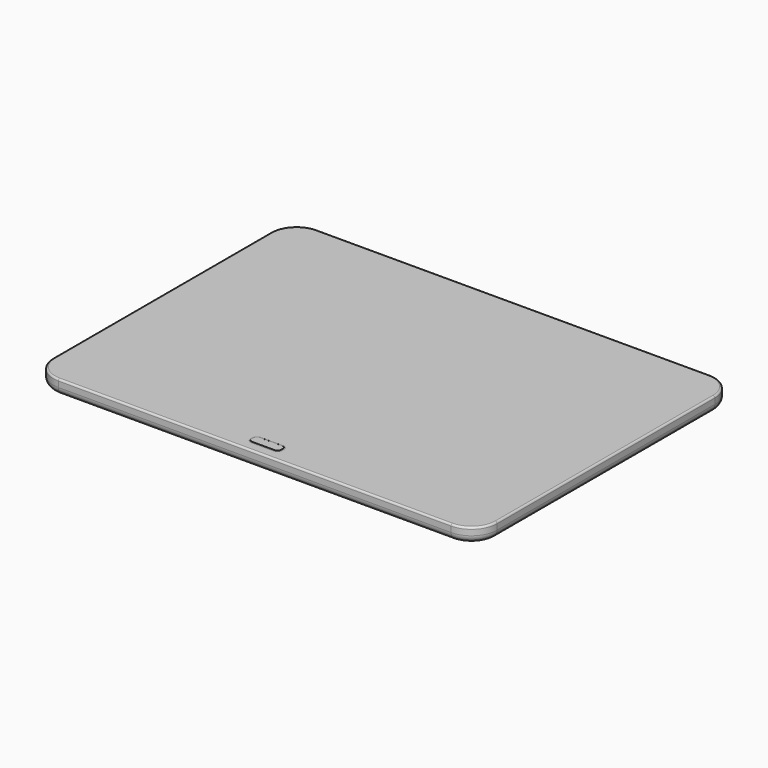
from build123d import *

# Parameters (mm, degrees)
F0_W         = 243
F0_H         = 177
F1_DEPTH     = 8.1
F2_R         = 14
F3_W         = 16.2
F3_H         = 5.2
F4_DEPTH     = 0.2
F5_R         = 2
F6_R         = 4
F7_T1_DEPTH  = 12.2
F7_T3_DEPTH  = 1.2
F7_T6_ANGLE  = 90
F7_T8_ANGLE  = 90
F7_T10_ANGLE = 90
F7_T12_ANGLE = 90
F7_T13_DEPTH = 215
F7_T15_DEPTH = 149
F7_T18_ANGLE = 90
F7_T20_ANGLE = 90
F7_T22_ANGLE = 90
F7_T24_ANGLE = 90


# Not quite as in the source:
# - a fillet or chamfer that OpenCascade refuses, or shapes differently, is made with other operations: its cross-section is extruded or revolved along the edge and cut away or added


with BuildPart() as f1:
    # F0 (on Top) → F1 (new body)
    with BuildSketch(Plane.XY):
        with Locations((0, 88.5)):
            Rectangle(F0_W, F0_H)
    extrude(amount=F1_DEPTH)

    # F2
    f2_edges = [f1.edges().sort_by_distance(p)[0] for p in [
        (-121.5, 0, 4.05),
        (121.5, 0, 4.05),
        (121.5, 177, 4.05),
        (-121.5, 177, 4.05),
    ]]
    fillet(f2_edges, radius=F2_R)

    # F3 (on face) → F4 (join)
    with BuildSketch(Plane.XY.offset(8.1)):
        with Locations((0, 8.6)):
            Rectangle(F3_W, F3_H)
    extrude(amount=F4_DEPTH)

    # F5
    f5_edges = [f1.edges().sort_by_distance(p)[0] for p in [
        (8.1, 6, 8.2),
        (8.1, 11.2, 8.2),
        (-8.1, 6, 8.2),
        (-8.1, 11.2, 8.2),
    ]]
    fillet(f5_edges, radius=F5_R)

    # F6
    f6_edges = [f1.edges().sort_by_distance(p)[0] for p in [
        (121.5, 88.5, 0),
        (0, 177, 0),
        (117.399495, 172.899495, 0),
        (-117.399495, 172.899495, 0),
        (-121.5, 88.5, 0),
        (117.399495, 4.100505, 0),
        (-117.399495, 4.100505, 0),
        (0, 0, 0),
    ]]
    fillet(f6_edges, radius=F6_R)

    # F7: fillet of radius 1 on 16 edges, made by hand

    # F7_s2 → F7_t1 (join)
    with BuildSketch(Plane.YZ.offset(-6.1)):
        with BuildLine():
            ThreePointArc((11.8, 8.1), (11.483772234, 8.1513167019), (11.2, 8.3))
            Line((11.2, 8.3), (11.2, 8.1))
            Line((11.2, 8.1), (11.8, 8.1))
        make_face()
        with BuildLine():
            ThreePointArc((5.4, 8.1), (5.716227766, 8.1513167019), (6, 8.3))
            Line((6, 8.3), (6, 8.1))
            Line((6, 8.1), (5.4, 8.1))
        make_face()
    extrude(amount=F7_T1_DEPTH)

    # F7_s4 → F7_t3 (join)
    with BuildSketch(Plane.XZ.offset(-9.2)):
        with BuildLine():
            ThreePointArc((8.7, 8.1), (8.383772234, 8.1513167019), (8.1, 8.3))
            Line((8.1, 8.3), (8.1, 8.1))
            Line((8.1, 8.1), (8.7, 8.1))
        make_face()
        with BuildLine():
            ThreePointArc((-8.7, 8.1), (-8.383772234, 8.1513167019), (-8.1, 8.3))
            Line((-8.1, 8.3), (-8.1, 8.1))
            Line((-8.1, 8.1), (-8.7, 8.1))
        make_face()
    extrude(amount=F7_T3_DEPTH)

    # F7_s5 → F7_t6 (revolve)
    with BuildSketch(Plane.YZ.offset(6.1)):
        with BuildLine():
            ThreePointArc((11.8, 8.1), (11.483772234, 8.1513167019), (11.2, 8.3))
            Line((11.2, 8.3), (11.2, 8.1))
            Line((11.2, 8.1), (11.8, 8.1))
        make_face()
    revolve(axis=Axis((6.1, 9.2, 8.1), (0, 0, -1)), revolution_arc=F7_T6_ANGLE)

    # F7_s7 → F7_t8 (revolve)
    with BuildSketch(Plane.YZ.offset(-6.1)):
        with BuildLine():
            ThreePointArc((11.8, 8.1), (11.483772234, 8.1513167019), (11.2, 8.3))
            Line((11.2, 8.3), (11.2, 8.1))
            Line((11.2, 8.1), (11.8, 8.1))
        make_face()
    revolve(axis=Axis((-6.1, 9.2, 8.1), (0, 0, 1)), revolution_arc=F7_T8_ANGLE)

    # F7_s9 → F7_t10 (revolve)
    with BuildSketch(Plane.YZ.offset(6.1)):
        with BuildLine():
            ThreePointArc((5.4, 8.1), (5.716227766, 8.1513167019), (6, 8.3))
            Line((6, 8.3), (6, 8.1))
            Line((6, 8.1), (5.4, 8.1))
        make_face()
    revolve(axis=Axis((6.1, 8, 8.1), (0, 0, 1)), revolution_arc=F7_T10_ANGLE)

    # F7_s11 → F7_t12 (revolve)
    with BuildSketch(Plane.XZ.offset(-8)):
        with BuildLine():
            ThreePointArc((-8.7, 8.1), (-8.383772234, 8.1513167019), (-8.1, 8.3))
            Line((-8.1, 8.3), (-8.1, 8.1))
            Line((-8.1, 8.1), (-8.7, 8.1))
        make_face()
    revolve(axis=Axis((-6.1, 8, 8.1), (0, 0, 1)), revolution_arc=F7_T12_ANGLE)

    # F7_s14 → F7_t13 (cut)
    with BuildSketch(Plane.YZ.offset(-107.5)):
        with BuildLine():
            ThreePointArc((177, 7.1), (176.7071067812, 7.8071067812), (176, 8.1))
            Line((176, 8.1), (177, 8.1))
            Line((177, 8.1), (177, 7.1))
        make_face()
        with BuildLine():
            ThreePointArc((1, 8.1), (0.2928932188, 7.8071067812), (0, 7.1))
            Line((0, 7.1), (0, 8.1))
            Line((0, 8.1), (1, 8.1))
        make_face()
    extrude(amount=F7_T13_DEPTH, mode=Mode.SUBTRACT)

    # F7_s16 → F7_t15 (cut)
    with BuildSketch(Plane.XZ.offset(-163)):
        with BuildLine():
            ThreePointArc((120.5, 8.1), (121.2071067812, 7.8071067812), (121.5, 7.1))
            Line((121.5, 7.1), (121.5, 8.1))
            Line((121.5, 8.1), (120.5, 8.1))
        make_face()
        with BuildLine():
            ThreePointArc((-120.5, 8.1), (-121.2071067812, 7.8071067812), (-121.5, 7.1))
            Line((-121.5, 7.1), (-121.5, 8.1))
            Line((-121.5, 8.1), (-120.5, 8.1))
        make_face()
    extrude(amount=F7_T15_DEPTH, mode=Mode.SUBTRACT)

    # F7_s17 → F7_t18 (revolve, cut)
    with BuildSketch(Plane.YZ.offset(107.5)):
        with BuildLine():
            ThreePointArc((177, 7.1), (176.7071067812, 7.8071067812), (176, 8.1))
            Line((176, 8.1), (177, 8.1))
            Line((177, 8.1), (177, 7.1))
        make_face()
    revolve(axis=Axis((107.5, 163, 8.1), (0, 0, -1)), revolution_arc=F7_T18_ANGLE, mode=Mode.SUBTRACT)

    # F7_s19 → F7_t20 (revolve, cut)
    with BuildSketch(Plane.YZ.offset(-107.5)):
        with BuildLine():
            ThreePointArc((176, 8.1), (176.7071067812, 7.8071067812), (177, 7.1))
            Line((177, 7.1), (177, 8.1))
            Line((177, 8.1), (176, 8.1))
        make_face()
    revolve(axis=Axis((-107.5, 163, 8.1), (0, 0, 1)), revolution_arc=F7_T20_ANGLE, mode=Mode.SUBTRACT)

    # F7_s21 → F7_t22 (revolve, cut)
    with BuildSketch(Plane.YZ.offset(107.5)):
        with BuildLine():
            ThreePointArc((1, 8.1), (0.2928932188, 7.8071067812), (0, 7.1))
            Line((0, 7.1), (0, 8.1))
            Line((0, 8.1), (1, 8.1))
        make_face()
    revolve(axis=Axis((107.5, 14, 8.1), (0, 0, 1)), revolution_arc=F7_T22_ANGLE, mode=Mode.SUBTRACT)

    # F7_s23 → F7_t24 (revolve, cut)
    with BuildSketch(Plane.XZ.offset(-14)):
        with BuildLine():
            ThreePointArc((-120.5, 8.1), (-121.2071067812, 7.8071067812), (-121.5, 7.1))
            Line((-121.5, 7.1), (-121.5, 8.1))
            Line((-121.5, 8.1), (-120.5, 8.1))
        make_face()
    revolve(axis=Axis((-107.5, 14, 8.1), (0, 0, 1)), revolution_arc=F7_T24_ANGLE, mode=Mode.SUBTRACT)


solid = f1.part
